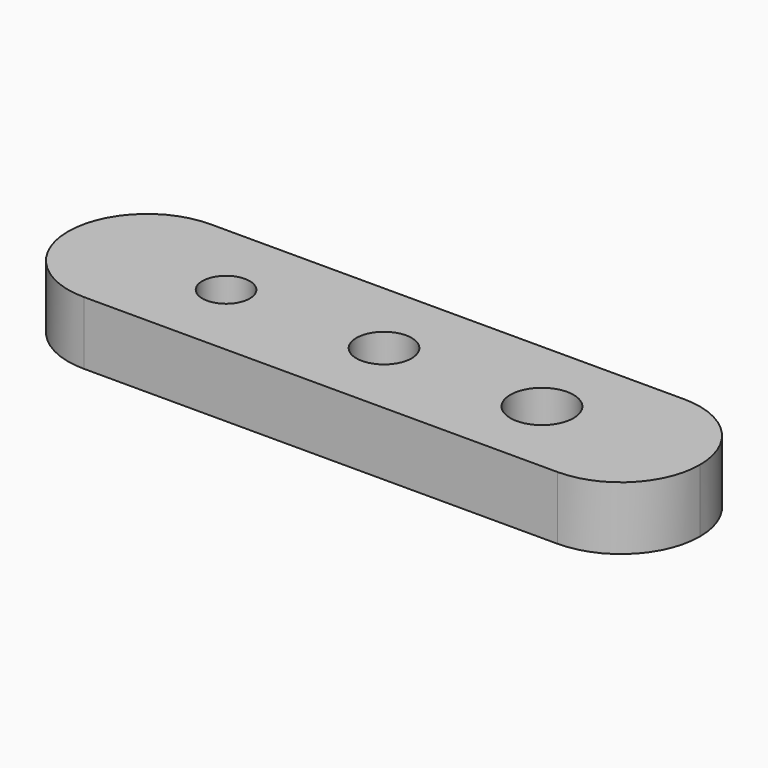
from build123d import *

# Parameters (mm, degrees)
F0_W     = 40
F0_H     = 10
F0_R     = 1.5
F0_R_2   = 1.75
F0_R_3   = 2
F1_DEPTH = 4
F2_R     = 4.99999


# Not quite as in the source:
# - a fillet or chamfer is up to 0.001 mm smaller than in the source, because OpenCascade refuses the exact size


with BuildPart() as f1:
    # F0 (on Top) → F1 (new body)
    with BuildSketch(Plane.XY):
        Rectangle(F0_W, F0_H)
        with Locations((-10, 0)):
            Circle(F0_R, mode=Mode.SUBTRACT)
        Circle(F0_R_2, mode=Mode.SUBTRACT)
        with Locations((10, 0)):
            Circle(F0_R_3, mode=Mode.SUBTRACT)
    extrude(amount=F1_DEPTH)

    # F2 (radius 5 in the source; OpenCascade refuses exactly that, so slightly less here)
    f2_edges = [f1.edges().sort_by_distance(p)[0] for p in [
        (-20, 5, 2),
        (-20, -5, 2),
        (20, -5, 2),
        (20, 5, 2),
    ]]
    fillet(f2_edges, radius=F2_R)


solid = f1.part
